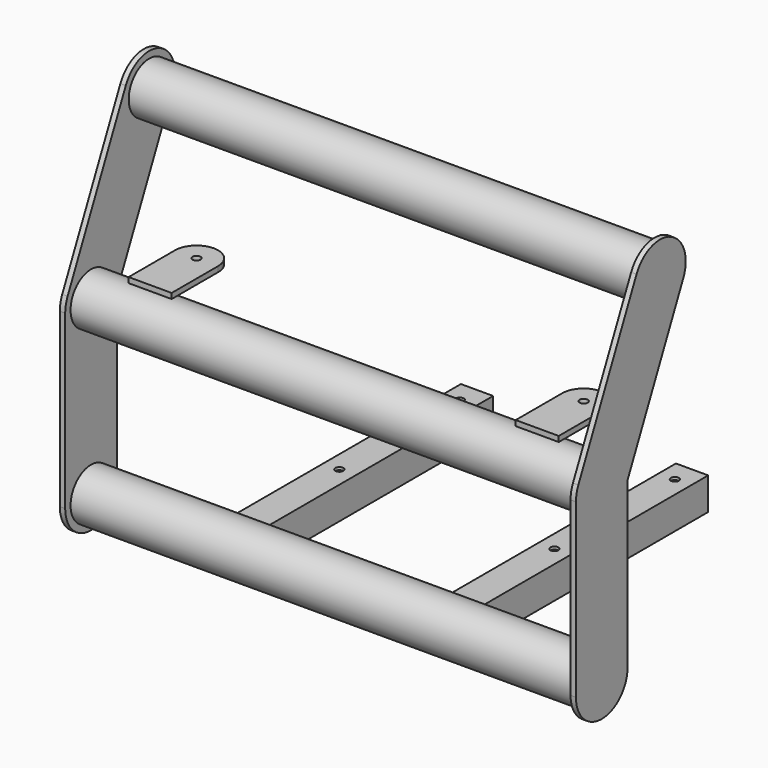
from build123d import *

# Parameters (mm, degrees)
F1_DEPTH  = 609.6
F2_W      = 596.9
F2_H      = 510.7920589639
F3_DEPTH  = 162.0770261002
F4_R      = 30.1625
F4_R_2    = 26.2509
F5_DEPTH  = 596.9
F6_R      = 30.1625
F6_R_2    = 26.2509
F7_DEPTH  = 596.9
F8_R      = 30.1625
F8_R_2    = 26.2509
F9_DEPTH  = 596.9
F10_W     = 38.1
F10_H     = 38.1
F10_W_2   = 31.75
F10_H_2   = 31.75
F11_DEPTH = 355.6
F12_R     = 30.1625
F13_DEPTH = 38.1
F14_R     = 4.7625
F15_DEPTH = 57.151
F17_W     = 50.8
F17_H     = 6.35
F18_DEPTH = 93.98
F19_R     = 25.39999
F20_R     = 4.7625
F21_DEPTH = 303.2135


# Not quite as in the source:
# - a fillet or chamfer is up to 0.001 mm smaller than in the source, because OpenCascade refuses the exact size


with BuildPart() as f1:
    # F0 (on Right) → F1 (new body)
    with BuildSketch(Plane.YZ):
        with BuildLine():
            ThreePointArc((-38.1, 0), (0, -38.1), (38.1, 0))
            ThreePointArc((38.1, 0), (0, 38.1), (-38.1, 0))
        make_face()
        with BuildLine():
            ThreePointArc((-38.1, 0), (0, 38.1), (38.1, 0))
            Line((38.1, 0), (38.1, 194.7534333533))
            Line((38.1, 194.7534333533), (34.5303266861, 187.0982442277))
            ThreePointArc((34.5303266861, 187.0982442277), (-8.246349291, 166.0031221287), (-38.1, 203.2))
            Line((-38.1, 203.2), (-38.1, 0))
        make_face()
        with BuildLine():
            Line((38.1, 203.2), (38.1, 194.7534333533))
            Line((38.1, 194.7534333533), (120.4063527863, 371.2599765055))
            ThreePointArc((120.4063527863, 371.2599765055), (69.7742703279, 352.8314055917), (51.3456994141, 403.4634880501))
            Line((51.3456994141, 403.4634880501), (-34.5303266861, 219.3017557723))
            ThreePointArc((-34.5303266861, 219.3017557723), (8.246349291, 240.3968778713), (38.1, 203.2))
        make_face()
        with BuildLine():
            Line((34.5303266861, 187.0982442277), (38.1, 194.7534333533))
            Line((38.1, 194.7534333533), (38.1, 203.2))
            ThreePointArc((38.1, 203.2), (37.1968778713, 194.953650709), (34.5303266861, 187.0982442277))
        make_face()
        with BuildLine():
            ThreePointArc((-34.5303266861, 219.3017557723), (-37.1968778713, 211.446349291), (-38.1, 203.2))
            ThreePointArc((-38.1, 203.2), (-8.246349291, 166.0031221287), (34.5303266861, 187.0982442277))
            ThreePointArc((34.5303266861, 187.0982442277), (37.1968778713, 194.953650709), (38.1, 203.2))
            ThreePointArc((38.1, 203.2), (8.246349291, 240.3968778713), (-34.5303266861, 219.3017557723))
        make_face()
        with BuildLine():
            ThreePointArc((51.3456994141, 403.4634880501), (69.7742703279, 352.8314055917), (120.4063527863, 371.2599765055))
            ThreePointArc((120.4063527863, 371.2599765055), (123.0729039715, 379.1153829868), (123.9760261002, 387.3617322778))
            ThreePointArc((123.9760261002, 387.3617322778), (94.1223753913, 424.5586101491), (51.3456994141, 403.4634880501))
        make_face()
    extrude(amount=F1_DEPTH)

    # F2 (on face) → F3 (cut, through all)
    with BuildSketch(Plane.XZ.offset(38.1)):
        with Locations((304.8, 191.896029482)):
            Rectangle(F2_W, F2_H)
    extrude(amount=-F3_DEPTH, mode=Mode.SUBTRACT)


with BuildPart() as f5:
    # F4 (on face) → F5 (new body)
    with BuildSketch(Plane.YZ.offset(6.35)):
        Circle(F4_R)
        Circle(F4_R_2, mode=Mode.SUBTRACT)
    extrude(amount=F5_DEPTH)


with BuildPart() as f7:
    # F6 (on face) → F7 (new body)
    with BuildSketch(Plane.YZ.offset(6.35)):
        with Locations((0, 203.2)):
            Circle(F6_R)
        with Locations((0, 203.2)):
            Circle(F6_R_2, mode=Mode.SUBTRACT)
    extrude(amount=F7_DEPTH)


with BuildPart() as f9:
    # F8 (on face) → F9 (new body)
    with BuildSketch(Plane.YZ.offset(6.35)):
        with Locations((85.8760261002, 387.3617322778)):
            Circle(F8_R)
        with Locations((85.8760261002, 387.3617322778)):
            Circle(F8_R_2, mode=Mode.SUBTRACT)
    extrude(amount=F9_DEPTH)


with BuildPart() as f11:
    # F10 (on Front) → F11 (new body)
    with BuildSketch(Plane.XZ):
        with Locations((-76.2, 0)):
            Rectangle(F10_W, F10_H)
        with Locations((-76.2, 0)):
            Rectangle(F10_W_2, F10_H_2, mode=Mode.SUBTRACT)
    extrude(amount=-F11_DEPTH)

    # F12 (on face) → F13 (cut)
    with BuildSketch(Plane.YZ.offset(-57.15)):
        Circle(F12_R)
    extrude(amount=-F13_DEPTH, mode=Mode.SUBTRACT)

    # F14 (on face) → F15 (cut, through all)
    with BuildSketch(Plane.XY.offset(19.05)):
        with Locations((-76.2, 330.2)):
            Circle(F14_R)
        with Locations((-76.2, 152.4)):
            Circle(F14_R)
    extrude(amount=-F15_DEPTH, mode=Mode.SUBTRACT)


with BuildPart() as f11_1:
    # F16: moved
    add(f11.part.moved(Location((508, 0, 0))))


with BuildPart() as f18:
    # F17 (on Front) → F18 (new body)
    with BuildSketch(Plane.XZ):
        with Locations((76.2, 261.9375)):
            Rectangle(F17_W, F17_H)
    extrude(amount=-F18_DEPTH)

    # F19 (radius 25.4 in the source; OpenCascade refuses exactly that, so slightly less here)
    f19_edges = [f18.edges().sort_by_distance(p)[0] for p in [
        (101.6, 93.98, 261.9375),
        (50.8, 93.98, 261.9375),
    ]]
    fillet(f19_edges, radius=F19_R)

    # F20 (on face) → F21 (cut, through all)
    with BuildSketch(Plane.XY.offset(265.1125)):
        with Locations((76.2, 68.58)):
            Circle(F20_R)
    extrude(amount=-F21_DEPTH, mode=Mode.SUBTRACT)


with BuildPart() as f22_1:
    # F22: copy of F18
    add(f18.part.moved(Location((457.2, 0, -25.4))))


with BuildPart() as f18_1:
    # F23: moved
    add(f18.part.moved(Location((0, 0, -25.4))))


with BuildPart() as f24_1:
    # F24: copy of F11
    add(f11_1.part.moved(Location((-254, 0, 0))))


solid = Compound([f1.part, f5.part, f7.part, f9.part, f11_1.part, f22_1.part, f18_1.part, f24_1.part])
